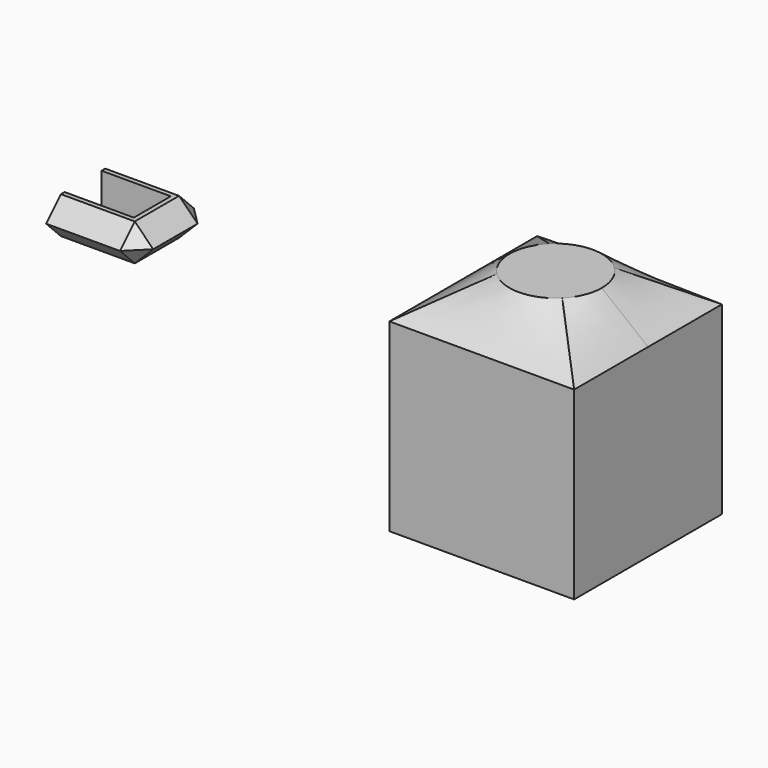
from build123d import *

# Parameters (mm, degrees)
F0_W      = 25.4
F0_H      = 25.4
F1_DEPTH  = 25.4
F1_FACE_W = 25.4
F1_FACE_H = 25.4
F3_R      = 6.35
F10_W     = 12.7
F10_H     = 5.08
F11_DEPTH = 12.7
F13_DEPTH = 5.08
F14_SIZE  = 2.53999


# Not quite as in the source:
# - a fillet or chamfer is up to 0.001 mm smaller than in the source, because OpenCascade refuses the exact size


with BuildPart() as f1:
    # F0 (on Top) → F1 (new body)
    with BuildSketch(Plane.XY):
        with Locations((12.7, 12.7)):
            Rectangle(F0_W, F0_H)
    extrude(amount=F1_DEPTH)

    # F1_face (on face) → F4 section 0
    with BuildSketch(Plane(origin=(12.7, 12.7, 25.4), x_dir=(1, 0, 0), z_dir=(0, 0, 1))):
        Rectangle(F1_FACE_W, F1_FACE_H)
    # F3 (on offset) → F4 section 1
    with BuildSketch(Plane.XY.offset(30.48)):
        with Locations((12.7, 12.7)):
            Circle(F3_R)
    loft()


with BuildPart() as f5_1:
    # F5: copy of F1
    add(f1.part)


with BuildPart() as f6_1:
    # F6: copy of F5_1
    add(f5_1.part)


with BuildPart() as f7_1:
    # F7: copy of F6_1
    add(f6_1.part)


with BuildPart() as f8_1:
    # F8: copy of F7_1
    add(f7_1.part)


with BuildPart() as f9_1:
    # F9: copy of F8_1
    add(f8_1.part)


with BuildPart() as f11:
    # F10 (on Right) → F11 (new body)
    with BuildSketch(Plane.YZ):
        with Locations((-52.6632983238, 61.217793389)):
            Rectangle(F10_W, F10_H)
    extrude(amount=F11_DEPTH)

    # F12 (on face) → F13 (cut)
    with BuildSketch(Plane(origin=(0, 0, 58.677793389), x_dir=(1, 0, 0), z_dir=(0, 0, -1))):
        Polygon((6.35, 55.8382983238), (0, 55.8382983238), (0, 52.6632983238), (0, 49.4882983238), (9.525, 49.4882983238), (9.525, 55.8382983238), align=None)
    extrude(amount=-F13_DEPTH, mode=Mode.SUBTRACT)

    # F14 (size 2.54 in the source; OpenCascade refuses exactly that, so slightly less here)
    f14_edges = [f11.edges().sort_by_distance(p)[0] for p in [
        (12.7, -59.013298, 61.217793),
        (12.7, -46.313298, 61.217793),
        (12.7, -52.663298, 58.677793),
        (12.7, -52.663298, 63.757793),
        (6.35, -46.313298, 58.677793),
        (6.35, -59.013298, 58.677793),
        (6.35, -59.013298, 63.757793),
        (6.35, -46.313298, 63.757793),
    ]]
    chamfer(f14_edges, length=F14_SIZE)


solid = Compound([f1.part, f5_1.part, f6_1.part, f7_1.part, f8_1.part, f9_1.part, f11.part])
